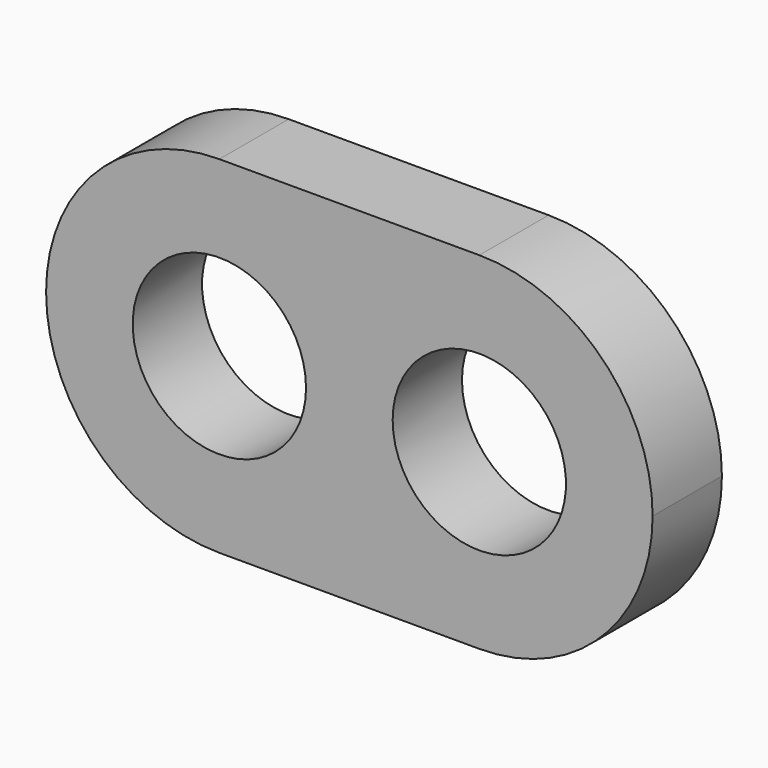
from build123d import *

# Parameters (mm, degrees)
F1_DEPTH = 25.4
F2_R     = 50.79999
F3_R     = 25.4
F4_DEPTH = 79.248


# Not quite as in the source:
# - a fillet or chamfer is up to 0.001 mm smaller than in the source, because OpenCascade refuses the exact size


with BuildPart() as f1:
    # F0 (on Front) → F1 (new body)
    with BuildSketch(Plane.XZ):
        with BuildLine():
            ThreePointArc((0, -50.8), (35.9210244843, -35.9210244843), (50.8, 0))
            ThreePointArc((50.8, 0), (35.9210244843, 35.9210244843), (0, 50.8))
            Line((0, 50.8), (0, -50.8))
        make_face()
        with BuildLine():
            ThreePointArc((0, 50.8), (35.9210244843, 35.9210244843), (50.8, 0))
            ThreePointArc((50.8, 0), (35.9210244843, -35.9210244843), (0, -50.8))
            Line((0, -50.8), (127, -50.8))
            Line((127, -50.8), (127, 50.8))
            Line((127, 50.8), (0, 50.8))
        make_face()
        with BuildLine():
            Line((0, -50.8), (0, 50.8))
            ThreePointArc((0, 50.8), (-50.8, 0), (0, -50.8))
        make_face()
    extrude(amount=F1_DEPTH)

    # F2 (radius 50.8 in the source; OpenCascade refuses exactly that, so slightly less here)
    f2_edges = [f1.edges().sort_by_distance(p)[0] for p in [
        (127, -12.7, 50.8),
        (127, -12.7, -50.8),
    ]]
    fillet(f2_edges, radius=F2_R)

    # F3 (on Front) → F4 (cut)
    with BuildSketch(Plane.XZ):
        Circle(F3_R)
    f4 = extrude(amount=F4_DEPTH, mode=Mode.SUBTRACT)

    # F7: F4 across plane
    add(f4.mirror(Plane.YZ.offset(38.1)), mode=Mode.SUBTRACT)


solid = f1.part
